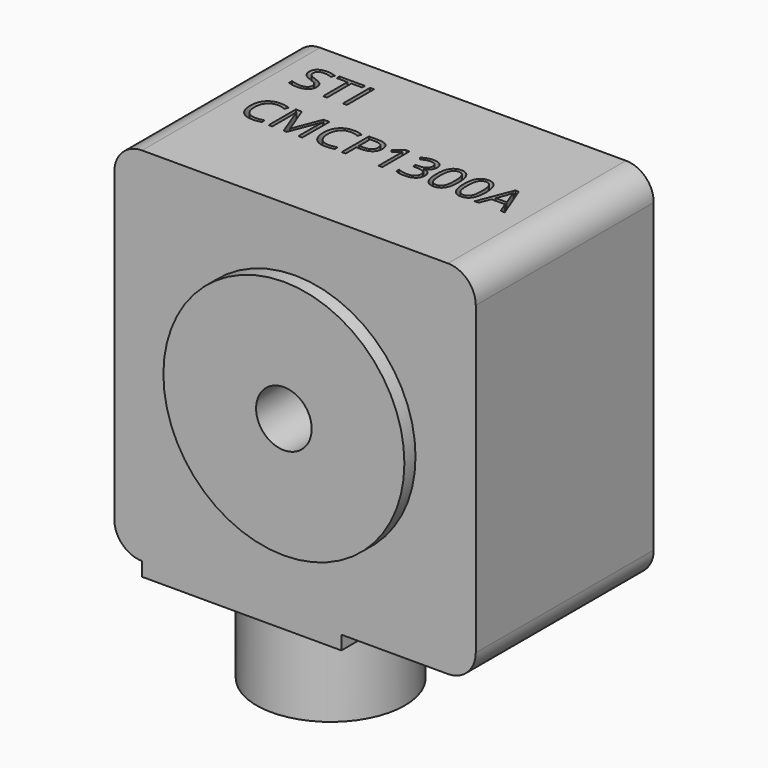
from build123d import *

# Parameters (mm, degrees)
F0_W          = 39
F0_H          = 39
F1_DEPTH      = 24
F2_R          = 3
F3_R          = 13
F4_DEPTH      = 1.5
F5_R          = 3
F6_DEPTH      = 25.501
F7_W          = 21.5
F7_H          = 24
F8_DEPTH      = 1.5
F9_R          = 8
F10_DEPTH     = 11
F11_TEXT_SIZE = 4.4571184036
F12_DEPTH     = 1
F13_TEXT_SIZE = 5.1398166559
F14_DEPTH     = 1


# Not quite as in the source:
# - Text() gives the source's letters only with a copy of the font that has no kerning and outlines rounded to 1/6400 em; it was checked with that copy


with BuildPart() as f1:
    # F0 (on Front) → F1 (new body)
    with BuildSketch(Plane.XZ):
        with Locations((19.5, 19.5)):
            Rectangle(F0_W, F0_H)
    extrude(amount=F1_DEPTH)

    # F2
    f2_edges = [f1.edges().sort_by_distance(p)[0] for p in [
        (0, -12, 39),
        (39, -12, 39),
        (39, -12, 0),
        (0, -12, 0),
    ]]
    fillet(f2_edges, radius=F2_R)

    # F3 (on face) → F4 (join)
    with BuildSketch(Plane.XZ.offset(24)):
        with Locations((19.5, 19.5)):
            Circle(F3_R)
    extrude(amount=F4_DEPTH)

    # F5 (on face) → F6 (cut, through all)
    with BuildSketch(Plane.XZ.offset(25.5)):
        with Locations((19.5, 19.5)):
            Circle(F5_R)
    extrude(amount=-F6_DEPTH, mode=Mode.SUBTRACT)

    # F7 (on face) → F8 (join)
    with BuildSketch(Plane(origin=(0, 0, 0), x_dir=(1, 0, 0), z_dir=(0, 0, -1))):
        with Locations((13.75, 12)):
            Rectangle(F7_W, F7_H)
    extrude(amount=F8_DEPTH)

    # F9 (on face) → F10 (join)
    with BuildSketch(Plane(origin=(0, 0, -1.5), x_dir=(1, 0, 0), z_dir=(0, 0, -1))):
        with Locations((13.75, 12)):
            Circle(F9_R)
    extrude(amount=F10_DEPTH)

    # F11 (on face) → F12 (cut)
    with BuildSketch(Plane(origin=(0, 0, 0), x_dir=(-1, 0, 0), z_dir=(0, 1, 0))):
        with Locations((-35.6683786958, 31.210731715)):
            Text('STI CMCP1300A', F11_TEXT_SIZE, font='Open Sans', text_align=(TextAlign.LEFT, TextAlign.BOTTOM))
    extrude(amount=-F12_DEPTH, mode=Mode.SUBTRACT)

    # F13 (on face) → F14 (cut)
    with BuildSketch(Plane.XY.offset(39)):
        with Locations((4.6965051442, -6.7486437038)):
            Text('STI', F13_TEXT_SIZE, font='Open Sans', text_align=(TextAlign.LEFT, TextAlign.BOTTOM))
        with Locations((4.6965051442, -13.7387943558)):
            Text('CMCP1300A', F13_TEXT_SIZE, font='Open Sans', text_align=(TextAlign.LEFT, TextAlign.BOTTOM))
    extrude(amount=-F14_DEPTH, mode=Mode.SUBTRACT)


solid = f1.part
